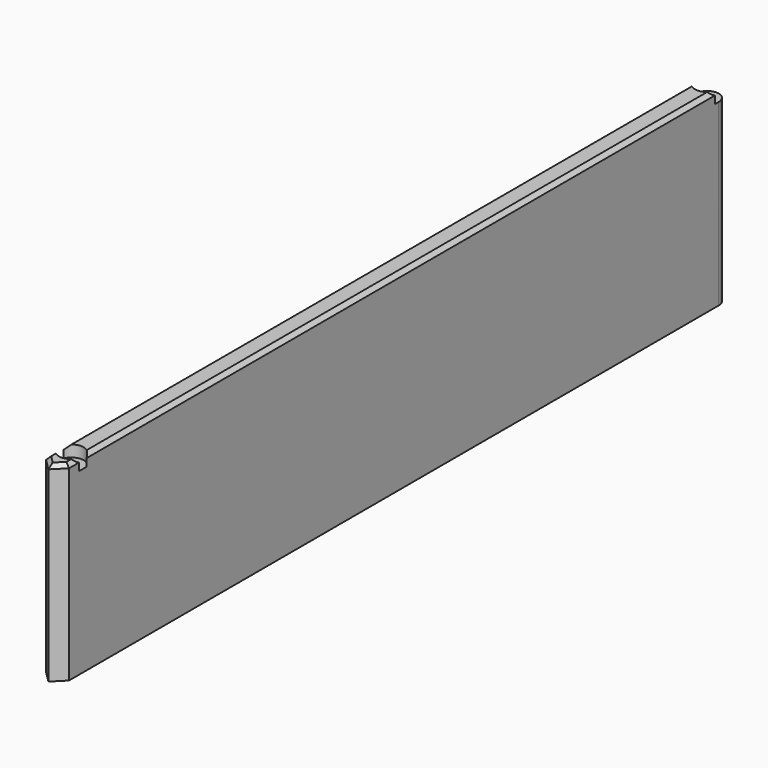
from build123d import *

# Parameters (mm, degrees)
F0_W     = 438
F0_H     = 100
F1_DEPTH = 12
F2_R     = 3
F3_DEPTH = 120
F4_START = 94
F2_R_2   = 6.5
F4_DEPTH = 6
F5_SIZE  = 5.99999
F6_SIZE  = 2
F7_R     = 5.99999


# Not quite as in the source:
# - a fillet or chamfer is up to 0.001 mm smaller than in the source, because OpenCascade refuses the exact size


with BuildPart() as f1:
    # F0 (on Right) → F1 (new body)
    with BuildSketch(Plane.YZ):
        with Locations((-219, 50)):
            Rectangle(F0_W, F0_H)
    extrude(amount=F1_DEPTH)

    # F2 (on Top) → F3 (cut)
    with BuildSketch(Plane.XY):
        with Locations((6, -422.9574446679)):
            Circle(F2_R)
        with Locations((6, -6)):
            Circle(F2_R)
    extrude(amount=F3_DEPTH, mode=Mode.SUBTRACT)

    # F2 (on Top) → F4 (cut)
    with BuildSketch(Plane.XY.offset(F4_START)):
        with Locations((6, -6)):
            Circle(F2_R_2)
        with Locations((6, -6)):
            Circle(F2_R, mode=Mode.SUBTRACT)
        with Locations((6, -422.9574446679)):
            Circle(F2_R_2)
        with Locations((6, -422.9574446679)):
            Circle(F2_R, mode=Mode.SUBTRACT)
    extrude(amount=F4_DEPTH, mode=Mode.SUBTRACT)

    # F5 (size 6 in the source; OpenCascade refuses exactly that, so slightly less here)
    f5_edges = [f1.edges().sort_by_distance(p)[0] for p in [
        (12, -438, 50),
        (0, -438, 50),
    ]]
    chamfer(f5_edges, length=F5_SIZE)

    # F6 (call 1 of 4: OpenCascade refuses the feature's edges together)
    f6_edges = [f1.edges().sort_by_distance(p)[0] for p in [
        (12, -428.728727, 100),
        (9.000005, -435.000005, 100),
    ]]
    chamfer(f6_edges, length=F6_SIZE)

    # F6#2 (call 2 of 4)
    f6_2_edges = [f1.edges().sort_by_distance(p)[0] for p in [
        (0, -428.728727, 100),
        (2.999995, -435.000005, 100),
    ]]
    chamfer(f6_2_edges, length=F6_SIZE)

    # F6#3 (call 3 of 4)
    f6_3_edges = [f1.edges().sort_by_distance(p)[0] for p in [
        (12, -214.478722, 100),
    ]]
    chamfer(f6_3_edges, length=F6_SIZE)

    # F6#4 (call 4 of 4)
    f6_4_edges = [f1.edges().sort_by_distance(p)[0] for p in [
        (0, -214.478722, 100),
    ]]
    chamfer(f6_4_edges, length=F6_SIZE)

    # F7 (radius 6 in the source; OpenCascade refuses exactly that, so slightly less here)
    f7_edges = [f1.edges().sort_by_distance(p)[0] for p in [
        (12, 0, 50),
        (0, 0, 50),
    ]]
    fillet(f7_edges, radius=F7_R)


solid = f1.part
